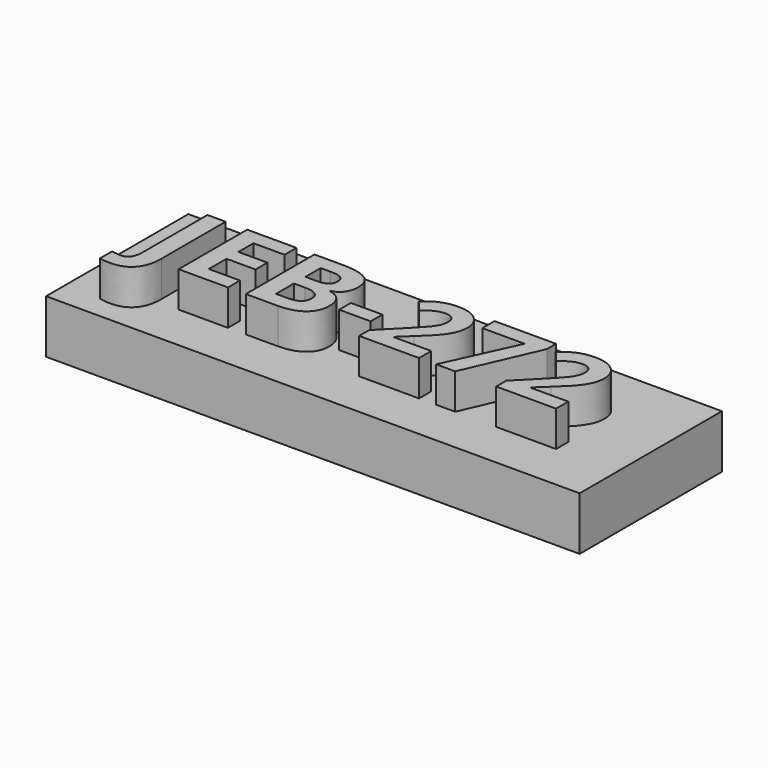
from build123d import *

# Parameters (mm, degrees)
F0_W         = 30
F0_H         = 10
F1_DEPTH     = 3
F2_TEXT_SIZE = 6.7487767842
F3_DEPTH     = 2


# Not quite as in the source:
# - Text() gives the source's letters only with a copy of the font that has no kerning and outlines rounded to 1/6400 em; it was checked with that copy


with BuildPart() as f1:
    # F0 (on Top) → F1 (new body)
    with BuildSketch(Plane.XY):
        Rectangle(F0_W, F0_H)
    extrude(amount=F1_DEPTH)

    # F2 (on face) → F3 (join)
    with BuildSketch(Plane.XY.offset(3)):
        with Locations((-12.5, -2.3591192846)):
            Text('JEB-272', F2_TEXT_SIZE, font='Open Sans', font_style=FontStyle.BOLD, text_align=(TextAlign.LEFT, TextAlign.BOTTOM))
    extrude(amount=F3_DEPTH)


solid = f1.part
